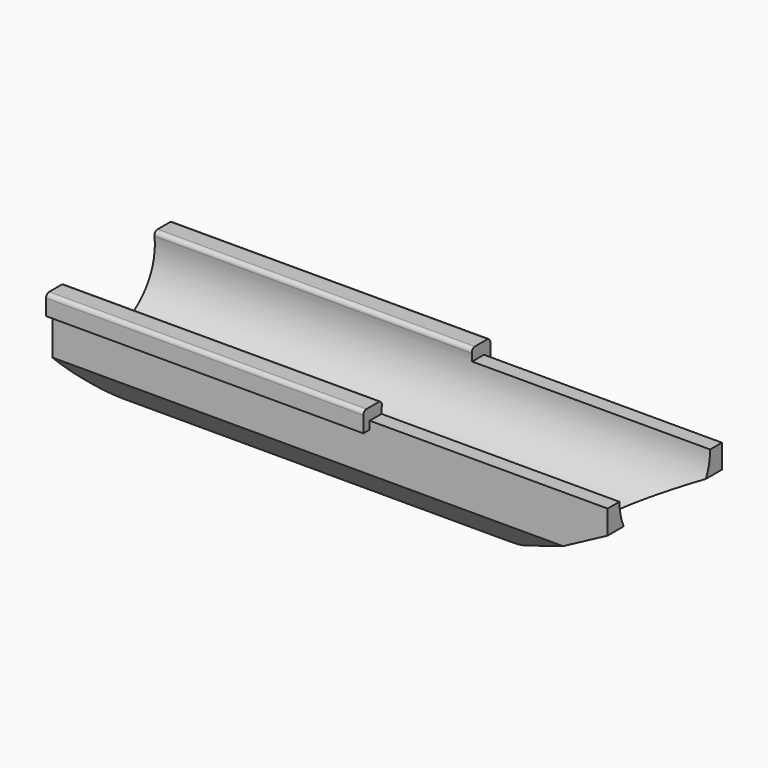
from build123d import *

# Parameters (mm, degrees)
F0_W        = 9
F0_H        = 11
F2_DEPTH    = 70
F1_W        = 10
F1_H        = 1
F1_H_2      = 1.5
F3_DEPTH    = 40
F4_D        = 14.2875
F5_T1_DEPTH = 95.6598919876
F6_SIZE     = 5
F7_T1_DEPTH = 14.25
F7_T3_DEPTH = 33
F8_R        = 0.5


# Not quite as in the source:
# - a fillet or chamfer that OpenCascade refuses, or shapes differently, is made with other operations: its cross-section is extruded or revolved along the edge and cut away or added
# - a length typed as a fraction of an inch, garbled in the dataset ("3 / 203.2 mm" for 3/8 in), is restored


with BuildPart() as f2:
    # F0 (on Right) → F2 (new body)
    with BuildSketch(Plane.YZ):
        with Locations((-4.5, -5.5)):
            Rectangle(F0_W, F0_H)
        with Locations((4.5, -5.5)):
            Rectangle(F0_W, F0_H)
    extrude(amount=F2_DEPTH)

    # F1 (on Right) → F3 (join)
    with BuildSketch(Plane.YZ):
        with Locations((-5, -0.5)):
            Rectangle(F1_W, F1_H)
        with Locations((5, -0.5)):
            Rectangle(F1_W, F1_H)
        with Locations((5, 0.75)):
            Rectangle(F1_W, F1_H_2)
        with Locations((-5, 0.75)):
            Rectangle(F1_W, F1_H_2)
    extrude(amount=F3_DEPTH)

    # F4 (through all)
    with Locations(Plane(origin=(0, 0, 0), x_dir=(0, 1, 0), z_dir=(-1, 0, 0))):
        with Locations((0, 0)):
            Hole(F4_D / 2)

    # F5: chamfer of 15 x 8 on 1 edges, made by hand

    # F5_s2 → F5_t1 (cut)
    with BuildSketch(Plane.XZ.offset(-47.8299459938)):
        Polygon((55, -11), (70, -3), (70, -11), align=None)
    extrude(amount=F5_T1_DEPTH, mode=Mode.SUBTRACT)

    # F6
    f6_edges = [f2.edges().sort_by_distance(p)[0] for p in [
        (27.5, 9, -11),
        (27.5, -9, -11),
    ]]
    chamfer(f6_edges, length=F6_SIZE)

    # F7: fillet of radius 5 on 2 edges, made by hand

    # F7_s2 → F7_t1 (cut)
    with BuildSketch(Plane.XZ.offset(-7.125)):
        with BuildLine():
            ThreePointArc((53.75, -11), (54.9626781252, -10.8507125007), (56.1029411765, -10.4117647059))
            Line((56.1029411765, -10.4117647059), (55, -11))
            Line((55, -11), (53.75, -11))
        make_face()
    extrude(amount=F7_T1_DEPTH, mode=Mode.SUBTRACT)

    # F7_s4 → F7_t3 (cut)
    with BuildSketch(Plane.XZ.offset(-16.5)):
        with BuildLine():
            ThreePointArc((0, -6), (1.4644660941, -9.5355339059), (5, -11))
            Line((5, -11), (0, -11))
            Line((0, -11), (0, -6))
        make_face()
    extrude(amount=F7_T3_DEPTH, mode=Mode.SUBTRACT)

    # F8
    f8_edges = [f2.edges().sort_by_distance(p)[0] for p in [
        (20, -10, 1.5),
        (20, 10, 1.5),
        (20, -6.984495, 1.5),
        (20, 6.984495, 1.5),
    ]]
    fillet(f8_edges, radius=F8_R)


solid = f2.part
